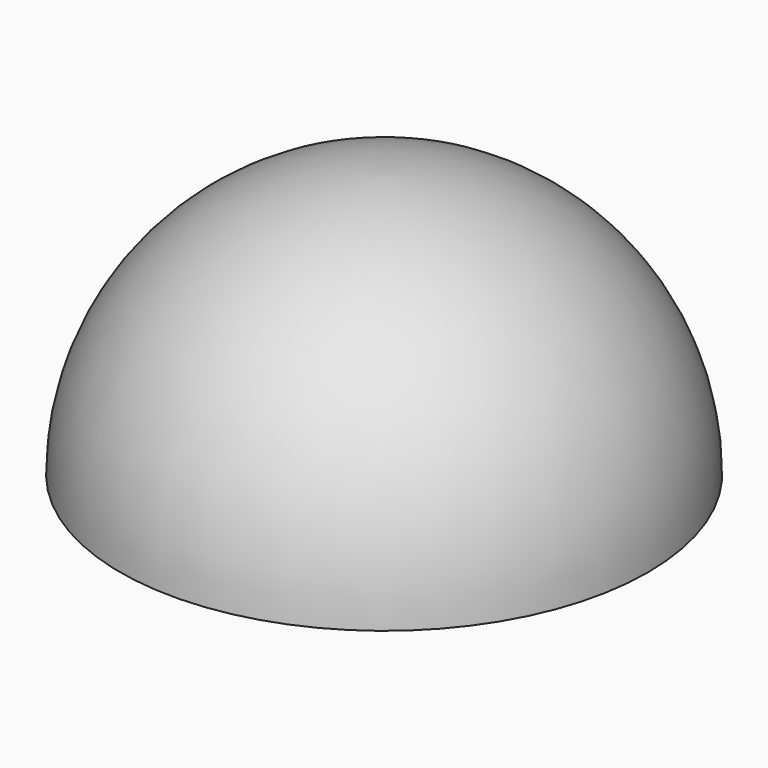
from build123d import *

# Parameters (mm, degrees)
F1_R     = 25.4
F2_DEPTH = 25.4
F3_R     = 25.39999
F4_R     = 16.1798
F5_DEPTH = 2.54


# Not quite as in the source:
# - a variable given as a bare number and used for a length is read in inches; the dataset says mm whatever the document's units were
# - a fillet or chamfer is up to 0.001 mm smaller than in the source, because OpenCascade refuses the exact size


with BuildPart() as f2:
    # F1 (on Top) → F2 (new body)
    with BuildSketch(Plane.XY):
        Circle(F1_R)
    extrude(amount=F2_DEPTH)

    # F3 (radius 25.4 in the source; OpenCascade refuses exactly that, so slightly less here)
    f3_edges = [f2.edges().sort_by_distance(p)[0] for p in [
        (-25.4, 0, 25.4),
    ]]
    fillet(f3_edges, radius=F3_R)

    # F4 (on face) → F5 (join)
    with BuildSketch(Plane(origin=(0, 0, 0), x_dir=(1, 0, 0), z_dir=(0, 0, -1))):
        Circle(F4_R)
    extrude(amount=F5_DEPTH)


solid = f2.part
